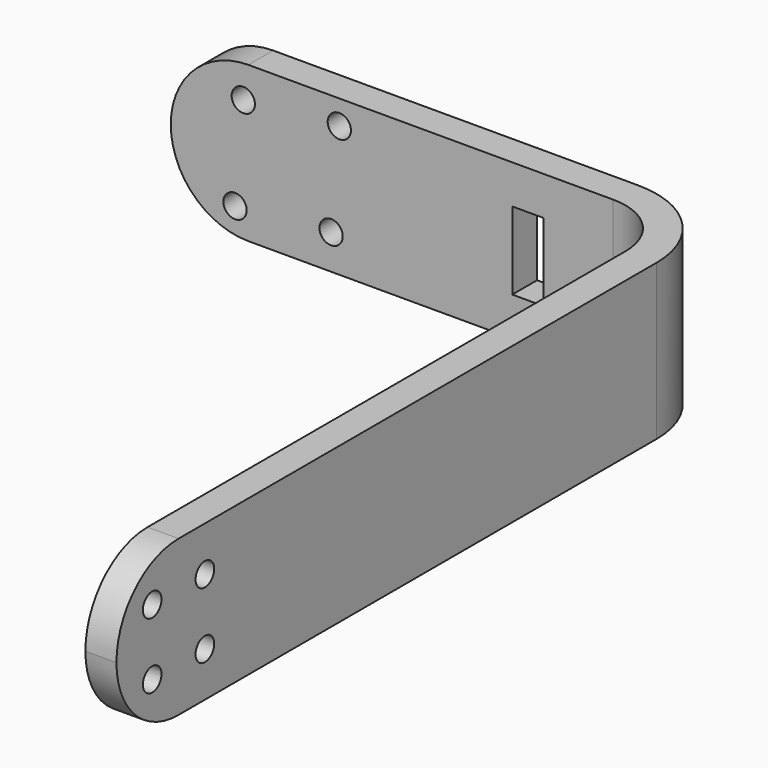
from build123d import *

# Parameters (mm, degrees)
F1_DEPTH = 20
F4_R     = 9.99999
F6_D     = 3
F2_W     = 4
F2_H     = 10
F7_DEPTH = 25
F8_D     = 3


# Not quite as in the source:
# - a fillet or chamfer is up to 0.001 mm smaller than in the source, because OpenCascade refuses the exact size
# - a feature names something its author has since deleted; it is built from what else it names


with BuildPart() as f1:
    # F0 (on Top) → F1 (new body)
    with BuildSketch(Plane.XY):
        with BuildLine():
            Line((0, 4), (0, 0))
            Line((0, 0), (57, 0))
            ThreePointArc((57, 0), (62.6568542495, -2.3431457505), (65, -8))
            Line((65, -8), (65, -95))
            Line((65, -95), (69, -95))
            Line((69, -95), (69, -8))
            ThreePointArc((69, -8), (65.4852813742, 0.4852813742), (57, 4))
            Line((57, 4), (0, 4))
        make_face()
    extrude(amount=F1_DEPTH)

    # F4 (radius 10 in the source; OpenCascade refuses exactly that, so slightly less here)
    f4_edges = [f1.edges().sort_by_distance(p)[0] for p in [
        (0, 2, 20),
        (0, 2, 0),
        (67, -95, 20),
        (67, -95, 0),
    ]]
    fillet(f4_edges, radius=F4_R)

    # F6 (through all)
    with Locations(Plane(origin=(65, 0, 0), x_dir=(0, -1, 0), z_dir=(-1, 0, 0))):
        with Locations((80.7573593129, 14.2426406871), (80.7573593129, 5.7573593129), (89.2426406871, 5.7573593129), (89.2426406871, 14.2426406871)):
            Hole(F6_D / 2)

    # F2 (on face) → F7 (cut)
    with BuildSketch(Plane.XZ):
        with Locations((46, 10)):
            Rectangle(F2_W, F2_H)
    extrude(amount=-F7_DEPTH, mode=Mode.SUBTRACT)

    # F8 (through all)
    with Locations(Plane.XZ):
        with Locations((8.2824855787, 3.4264645687), (21.7175144213, 16.8614934112), (20.6568542495, 4.4871247404), (9.3431457505, 15.8008332394)):
            Hole(F8_D / 2)


solid = f1.part
